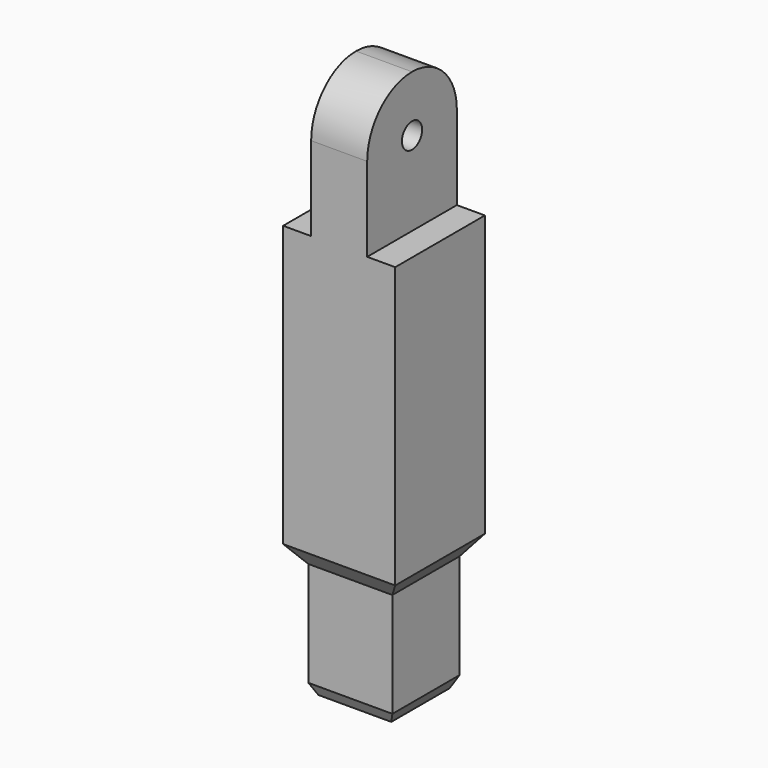
from build123d import *

# Parameters (mm, degrees)
F0_W           = 20
F0_H           = 20
F1_DEPTH       = 4
F2_W           = 10
F2_H           = 20
F3_DEPTH       = 25
F4_R           = 2.25
F5_DEPTH       = 15.001
F6_W           = 20
F6_H           = 20
F6_W_2         = 16
F6_H_2         = 16
F7_DEPTH       = 50
F8_W           = 16
F8_H           = 16
F8_W_2         = 12
F8_H_2         = 12
F9_DEPTH       = 20
F10_W          = 15
F10_H          = 15
F10_W_2        = 12
F10_H_2        = 12
F11_DEPTH      = 20
F12_T4_DEPTH   = 40.6455806409
F12_T10_DEPTH  = 40.6455806409
F12_T16_DEPTH  = 40.6455806409
F12_T23_DEPTH  = 40.6455806409
F12_T29_DEPTH  = 40.6455806409
F12_T35_DEPTH  = 40.6455806409
F12_T41_DEPTH  = 40.6455806409
F12_T47_DEPTH  = 40.6455806409
F12_T54_DEPTH  = 40.6455806409
F12_T60_DEPTH  = 40.6455806409
F12_T66_DEPTH  = 40.6455806409
F12_T72_DEPTH  = 40.6455806409
F12_T78_DEPTH  = 40.6455806409
F12_T85_DEPTH  = 40.6455806409
F12_T91_DEPTH  = 40.6455806409
F12_T97_DEPTH  = 40.6455806409
F12_T103_DEPTH = 40.6455806409
F12_T109_DEPTH = 40.6455806409
F12_T116_DEPTH = 40.6455806409
F12_T122_DEPTH = 40.6455806409
F13_SIZE2      = 2
F13_SIZE       = 1


# Not quite as in the source:
# - a fillet or chamfer that OpenCascade refuses, or shapes differently, is made with other operations: its cross-section is extruded or revolved along the edge and cut away or added


with BuildPart() as f1:
    # F0 (on Top) → F1 (new body)
    with BuildSketch(Plane.XY):
        Rectangle(F0_W, F0_H)
    extrude(amount=F1_DEPTH)

    # F2 (on face) → F3 (join)
    with BuildSketch(Plane.XY.offset(4)):
        Rectangle(F2_W, F2_H)
    extrude(amount=F3_DEPTH)

    # F4 (on face) → F5 (cut, through all)
    with BuildSketch(Plane.YZ.offset(5)):
        with BuildLine():
            ThreePointArc((-10, 19), (-7.0710678119, 26.0710678119), (0, 29))
            Line((0, 29), (-10, 29))
            Line((-10, 29), (-10, 19))
        make_face()
        with BuildLine():
            ThreePointArc((0, 29), (7.0710678119, 26.0710678119), (10, 19))
            Line((10, 19), (10, 29))
            Line((10, 29), (0, 29))
        make_face()
        with Locations((0, 19)):
            Circle(F4_R)
    extrude(amount=-F5_DEPTH, mode=Mode.SUBTRACT)

    # F6 (on face) → F7 (join)
    with BuildSketch(Plane(origin=(0, 0, 0), x_dir=(1, 0, 0), z_dir=(0, 0, -1))):
        Rectangle(F6_W, F6_H)
        Rectangle(F6_W_2, F6_H_2, mode=Mode.SUBTRACT)
    extrude(amount=F7_DEPTH)

    # F8 (on face) → F9 (join)
    with BuildSketch(Plane(origin=(0, 0, -50), x_dir=(1, 0, 0), z_dir=(0, 0, -1))):
        Rectangle(F8_W, F8_H)
        Rectangle(F8_W_2, F8_H_2, mode=Mode.SUBTRACT)
    extrude(amount=-F9_DEPTH)

    # F10 (on face) → F11 (join)
    with BuildSketch(Plane(origin=(0, 0, -50), x_dir=(1, 0, 0), z_dir=(0, 0, -1))):
        Rectangle(F10_W, F10_H)
        Rectangle(F10_W_2, F10_H_2, mode=Mode.SUBTRACT)
    extrude(amount=F11_DEPTH)

    # F12: chamfer of 3 x 4 on 4 edges, made by hand


with BuildPart() as f12_tool2:
    # F12_s3 → F12_t4 (new body)
    with BuildSketch(Plane.YZ.offset(20.3227903205)):
        Polygon((-7, -50), (-10, -46), (-10, -50), align=None)
    extrude(amount=-F12_T4_DEPTH)

    split(bisect_by=Plane.XZ.offset(7.5), keep=Keep.BOTTOM)

    split(bisect_by=Plane.YZ.offset(7.5), keep=Keep.TOP)


with BuildPart() as f1_1:
    add(f1.part)

    # F12_t1: cut F12_tool2
    add(f12_tool2.part, mode=Mode.SUBTRACT)


with BuildPart() as f12_tool8:
    # F12_s9 → F12_t10 (new body)
    with BuildSketch(Plane.YZ.offset(20.3227903205)):
        Polygon((-7, -50), (-10, -46), (-10, -50), align=None)
    extrude(amount=-F12_T10_DEPTH)

    split(bisect_by=Plane.XZ.offset(7.5), keep=Keep.TOP)

    split(bisect_by=Plane.YZ.offset(7.5), keep=Keep.TOP)


with BuildPart() as f1_2:
    add(f1_1.part)

    # F12_t7: cut F12_tool8
    add(f12_tool8.part, mode=Mode.SUBTRACT)


with BuildPart() as f12_tool14:
    # F12_s15 → F12_t16 (new body)
    with BuildSketch(Plane.YZ.offset(20.3227903205)):
        Polygon((-7, -50), (-10, -46), (-10, -50), align=None)
    extrude(amount=-F12_T16_DEPTH)

    split(bisect_by=Plane.XZ.offset(7.5), keep=Keep.TOP)

    split(bisect_by=Plane.YZ.offset(-7.5), keep=Keep.TOP)

    split(bisect_by=Plane.YZ.offset(7.5), keep=Keep.BOTTOM)


with BuildPart() as f1_3:
    add(f1_2.part)

    # F12_t13: cut F12_tool14
    add(f12_tool14.part, mode=Mode.SUBTRACT)


with BuildPart() as f12_tool21:
    # F12_s22 → F12_t23 (new body)
    with BuildSketch(Plane.YZ.offset(20.3227903205)):
        Polygon((-7, -50), (-10, -46), (-10, -50), align=None)
    extrude(amount=-F12_T23_DEPTH)

    split(bisect_by=Plane.XZ.offset(7.5), keep=Keep.BOTTOM)

    split(bisect_by=Plane.YZ.offset(-7.5), keep=Keep.BOTTOM)


with BuildPart() as f1_4:
    add(f1_3.part)

    # F12_t20: cut F12_tool21
    add(f12_tool21.part, mode=Mode.SUBTRACT)


with BuildPart() as f12_tool27:
    # F12_s28 → F12_t29 (new body)
    with BuildSketch(Plane.YZ.offset(20.3227903205)):
        Polygon((-7, -50), (-10, -46), (-10, -50), align=None)
    extrude(amount=-F12_T29_DEPTH)

    split(bisect_by=Plane.XZ.offset(7.5), keep=Keep.TOP)

    split(bisect_by=Plane.YZ.offset(-7.5), keep=Keep.BOTTOM)


with BuildPart() as f1_5:
    add(f1_4.part)

    # F12_t26: cut F12_tool27
    add(f12_tool27.part, mode=Mode.SUBTRACT)


with BuildPart() as f12_tool33:
    # F12_s34 → F12_t35 (new body)
    with BuildSketch(Plane.XZ.offset(-20.3227903205)):
        Polygon((10, -46), (7, -50), (10, -50), align=None)
    extrude(amount=F12_T35_DEPTH)

    split(bisect_by=Plane.XZ.offset(-7.5), keep=Keep.BOTTOM)

    split(bisect_by=Plane.YZ.offset(7.5), keep=Keep.TOP)


with BuildPart() as f1_6:
    add(f1_5.part)

    # F12_t32: cut F12_tool33
    add(f12_tool33.part, mode=Mode.SUBTRACT)


with BuildPart() as f12_tool39:
    # F12_s40 → F12_t41 (new body)
    with BuildSketch(Plane.XZ.offset(-20.3227903205)):
        Polygon((10, -46), (7, -50), (10, -50), align=None)
    extrude(amount=F12_T41_DEPTH)

    split(bisect_by=Plane.XZ.offset(-7.5), keep=Keep.BOTTOM)

    split(bisect_by=Plane.YZ.offset(7.5), keep=Keep.BOTTOM)


with BuildPart() as f1_7:
    add(f1_6.part)

    # F12_t38: cut F12_tool39
    add(f12_tool39.part, mode=Mode.SUBTRACT)


with BuildPart() as f12_tool45:
    # F12_s46 → F12_t47 (new body)
    with BuildSketch(Plane.XZ.offset(-20.3227903205)):
        Polygon((10, -46), (7, -50), (10, -50), align=None)
    extrude(amount=F12_T47_DEPTH)

    split(bisect_by=Plane.XZ.offset(7.5), keep=Keep.BOTTOM)

    split(bisect_by=Plane.XZ.offset(-7.5), keep=Keep.TOP)

    split(bisect_by=Plane.YZ.offset(7.5), keep=Keep.TOP)


with BuildPart() as f1_8:
    add(f1_7.part)

    # F12_t44: cut F12_tool45
    add(f12_tool45.part, mode=Mode.SUBTRACT)


with BuildPart() as f12_tool52:
    # F12_s53 → F12_t54 (new body)
    with BuildSketch(Plane.XZ.offset(-20.3227903205)):
        Polygon((10, -46), (7, -50), (10, -50), align=None)
    extrude(amount=F12_T54_DEPTH)

    split(bisect_by=Plane.XZ.offset(7.5), keep=Keep.TOP)

    split(bisect_by=Plane.YZ.offset(7.5), keep=Keep.TOP)


with BuildPart() as f1_9:
    add(f1_8.part)

    # F12_t51: cut F12_tool52
    add(f12_tool52.part, mode=Mode.SUBTRACT)


with BuildPart() as f12_tool58:
    # F12_s59 → F12_t60 (new body)
    with BuildSketch(Plane.XZ.offset(-20.3227903205)):
        Polygon((10, -46), (7, -50), (10, -50), align=None)
    extrude(amount=F12_T60_DEPTH)

    split(bisect_by=Plane.XZ.offset(7.5), keep=Keep.TOP)

    split(bisect_by=Plane.YZ.offset(7.5), keep=Keep.BOTTOM)


with BuildPart() as f1_10:
    add(f1_9.part)

    # F12_t57: cut F12_tool58
    add(f12_tool58.part, mode=Mode.SUBTRACT)


with BuildPart() as f12_tool64:
    # F12_s65 → F12_t66 (new body)
    with BuildSketch(Plane.XZ.offset(20.3227903205)):
        Polygon((-7, -50), (-10, -46), (-10, -50), align=None)
    extrude(amount=-F12_T66_DEPTH)

    split(bisect_by=Plane.XZ.offset(7.5), keep=Keep.TOP)

    split(bisect_by=Plane.YZ.offset(-7.5), keep=Keep.TOP)


with BuildPart() as f1_11:
    add(f1_10.part)

    # F12_t63: cut F12_tool64
    add(f12_tool64.part, mode=Mode.SUBTRACT)


with BuildPart() as f12_tool70:
    # F12_s71 → F12_t72 (new body)
    with BuildSketch(Plane.XZ.offset(20.3227903205)):
        Polygon((-7, -50), (-10, -46), (-10, -50), align=None)
    extrude(amount=-F12_T72_DEPTH)

    split(bisect_by=Plane.XZ.offset(7.5), keep=Keep.TOP)

    split(bisect_by=Plane.YZ.offset(-7.5), keep=Keep.BOTTOM)


with BuildPart() as f1_12:
    add(f1_11.part)

    # F12_t69: cut F12_tool70
    add(f12_tool70.part, mode=Mode.SUBTRACT)


with BuildPart() as f12_tool76:
    # F12_s77 → F12_t78 (new body)
    with BuildSketch(Plane.XZ.offset(20.3227903205)):
        Polygon((-7, -50), (-10, -46), (-10, -50), align=None)
    extrude(amount=-F12_T78_DEPTH)

    split(bisect_by=Plane.XZ.offset(7.5), keep=Keep.BOTTOM)

    split(bisect_by=Plane.YZ.offset(-7.5), keep=Keep.BOTTOM)

    split(bisect_by=Plane.XZ.offset(-7.5), keep=Keep.TOP)


with BuildPart() as f1_13:
    add(f1_12.part)

    # F12_t75: cut F12_tool76
    add(f12_tool76.part, mode=Mode.SUBTRACT)


with BuildPart() as f12_tool83:
    # F12_s84 → F12_t85 (new body)
    with BuildSketch(Plane.XZ.offset(20.3227903205)):
        Polygon((-7, -50), (-10, -46), (-10, -50), align=None)
    extrude(amount=-F12_T85_DEPTH)

    split(bisect_by=Plane.YZ.offset(-7.5), keep=Keep.TOP)

    split(bisect_by=Plane.XZ.offset(-7.5), keep=Keep.BOTTOM)


with BuildPart() as f1_14:
    add(f1_13.part)

    # F12_t82: cut F12_tool83
    add(f12_tool83.part, mode=Mode.SUBTRACT)


with BuildPart() as f12_tool89:
    # F12_s90 → F12_t91 (new body)
    with BuildSketch(Plane.XZ.offset(20.3227903205)):
        Polygon((-7, -50), (-10, -46), (-10, -50), align=None)
    extrude(amount=-F12_T91_DEPTH)

    split(bisect_by=Plane.YZ.offset(-7.5), keep=Keep.BOTTOM)

    split(bisect_by=Plane.XZ.offset(-7.5), keep=Keep.BOTTOM)


with BuildPart() as f1_15:
    add(f1_14.part)

    # F12_t88: cut F12_tool89
    add(f12_tool89.part, mode=Mode.SUBTRACT)


with BuildPart() as f12_tool95:
    # F12_s96 → F12_t97 (new body)
    with BuildSketch(Plane.YZ.offset(-20.3227903205)):
        Polygon((7, -50), (10, -46), (10, -50), align=None)
    extrude(amount=F12_T97_DEPTH)

    split(bisect_by=Plane.YZ.offset(-7.5), keep=Keep.BOTTOM)

    split(bisect_by=Plane.XZ.offset(-7.5), keep=Keep.TOP)


with BuildPart() as f1_16:
    add(f1_15.part)

    # F12_t94: cut F12_tool95
    add(f12_tool95.part, mode=Mode.SUBTRACT)


with BuildPart() as f12_tool101:
    # F12_s102 → F12_t103 (new body)
    with BuildSketch(Plane.YZ.offset(-20.3227903205)):
        Polygon((7, -50), (10, -46), (10, -50), align=None)
    extrude(amount=F12_T103_DEPTH)

    split(bisect_by=Plane.YZ.offset(-7.5), keep=Keep.BOTTOM)

    split(bisect_by=Plane.XZ.offset(-7.5), keep=Keep.BOTTOM)


with BuildPart() as f1_17:
    add(f1_16.part)

    # F12_t100: cut F12_tool101
    add(f12_tool101.part, mode=Mode.SUBTRACT)


with BuildPart() as f12_tool107:
    # F12_s108 → F12_t109 (new body)
    with BuildSketch(Plane.YZ.offset(-20.3227903205)):
        Polygon((7, -50), (10, -46), (10, -50), align=None)
    extrude(amount=F12_T109_DEPTH)

    split(bisect_by=Plane.YZ.offset(-7.5), keep=Keep.TOP)

    split(bisect_by=Plane.XZ.offset(-7.5), keep=Keep.BOTTOM)

    split(bisect_by=Plane.YZ.offset(7.5), keep=Keep.BOTTOM)


with BuildPart() as f1_18:
    add(f1_17.part)

    # F12_t106: cut F12_tool107
    add(f12_tool107.part, mode=Mode.SUBTRACT)


with BuildPart() as f12_tool114:
    # F12_s115 → F12_t116 (new body)
    with BuildSketch(Plane.YZ.offset(-20.3227903205)):
        Polygon((7, -50), (10, -46), (10, -50), align=None)
    extrude(amount=F12_T116_DEPTH)

    split(bisect_by=Plane.XZ.offset(-7.5), keep=Keep.TOP)

    split(bisect_by=Plane.YZ.offset(7.5), keep=Keep.TOP)


with BuildPart() as f1_19:
    add(f1_18.part)

    # F12_t113: cut F12_tool114
    add(f12_tool114.part, mode=Mode.SUBTRACT)


with BuildPart() as f12_tool120:
    # F12_s121 → F12_t122 (new body)
    with BuildSketch(Plane.YZ.offset(-20.3227903205)):
        Polygon((7, -50), (10, -46), (10, -50), align=None)
    extrude(amount=F12_T122_DEPTH)

    split(bisect_by=Plane.XZ.offset(-7.5), keep=Keep.BOTTOM)

    split(bisect_by=Plane.YZ.offset(7.5), keep=Keep.TOP)


with BuildPart() as f1_20:
    add(f1_19.part)

    # F12_t119: cut F12_tool120
    add(f12_tool120.part, mode=Mode.SUBTRACT)

    # F13
    f13_edges = [f1_20.edges().sort_by_distance(p)[0] for p in [
        (0, -7.5, -70),
        (7.5, 0, -70),
        (-7.5, 0, -70),
        (0, 7.5, -70),
    ]]
    f13_side = f1_20.faces().sort_by_distance((0, -7.287868, -70))[0]
    chamfer(f13_edges, length=F13_SIZE, length2=F13_SIZE2, reference=f13_side)


with BuildPart() as f14_1:
    # F14: copy of F1
    add(f1_20.part)


solid = Compound([f1_20.part, f14_1.part])
